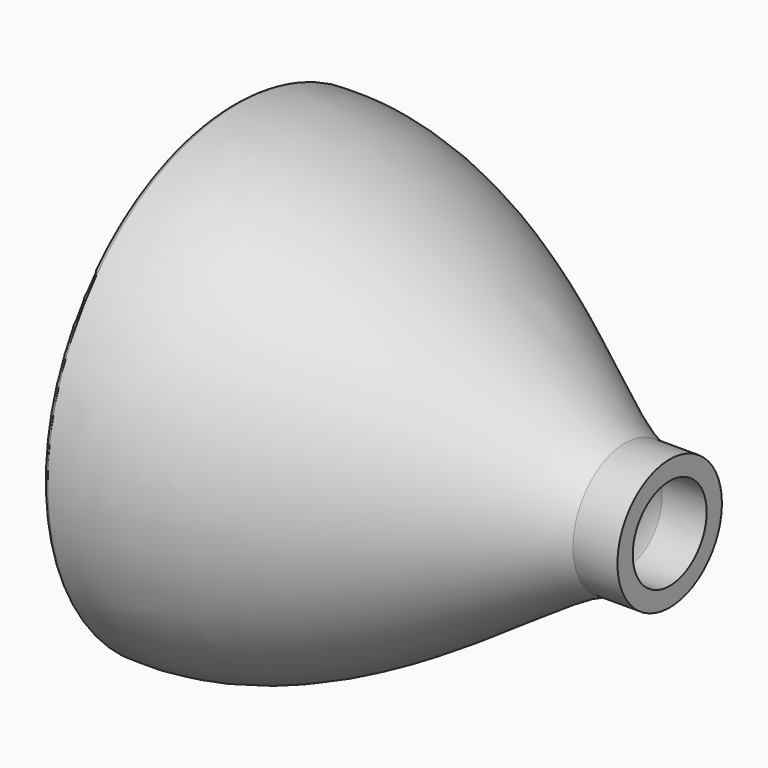
from build123d import *


# Not quite as in the source:
# - ends of sketch curves that miss each other by under 0.0002 mm in the source are joined
# - the dataset's text gives a spline's control points without its knots; the knots are read off the source's solid


with BuildPart() as f1:
    # F0 (on Top) → F1 (revolve)
    with BuildSketch(Plane.XY):
        Polygon((91.3116050863, 22.3759908215), (76.0716050863, 22.3759908215), (76.0716050863, 16.0226677732), (76.0716050863, 15.8381145447), (91.3116050863, 15.8381145447), align=None)
        with BuildLine():
            Line((76.0716050863, 16.0226677732), (76.0716050863, 22.3759908215))
            add(Edge.make_bspline(
                [(-56.4722613609, 81.6401132205), (-52.6798548628, 81.7974523925), (-45.1427955186, 81.6082252704), (-30.3507258747, 79.4792224524), (-12.5126860956, 74.0390077394), (7.5999931638, 64.5670910238), (26.1953157898, 53.5418439599), (40.1996337275, 44.1849486662), (50.3368797082, 37.2762913548), (57.3522822479, 32.5567032312), (63.7139533786, 28.4764684874), (69.3281338193, 25.2178951661), (73.2614295087, 23.3436374263), (75.296096269, 22.6107511928), (75.9695894554, 22.4060960407), (76.0716050863, 22.3759908215)],
                knots=[0, 0, 0, 0, 0.0625, 0.125, 0.25, 0.375, 0.5, 0.625, 0.6875, 0.75, 0.8125, 0.875, 0.9375, 0.96875, 0.974461933, 0.974461933, 0.974461933, 0.974461933], degree=3))
            ThreePointArc((-56.4722613609, 81.6401132205), (-58.7091129412, 78.369579758), (-56.2090393346, 75.2955716118))
            add(Edge.make_bspline(
                [(-56.2090393346, 75.2955716118), (0, 77.627569437), (53.4257777035, 20.3464794904), (76.0716050863, 15.8381145447)],
                knots=[0, 0, 0, 0, 145.0288181338, 145.0288181338, 145.0288181338, 145.0288181338], degree=3))
            Line((76.0716050863, 15.8381145447), (76.0716050863, 16.0226677732))
        make_face()
    revolve(axis=Axis((4.5482069254, 0, 0), (1, 0, 0)))


solid = f1.part
